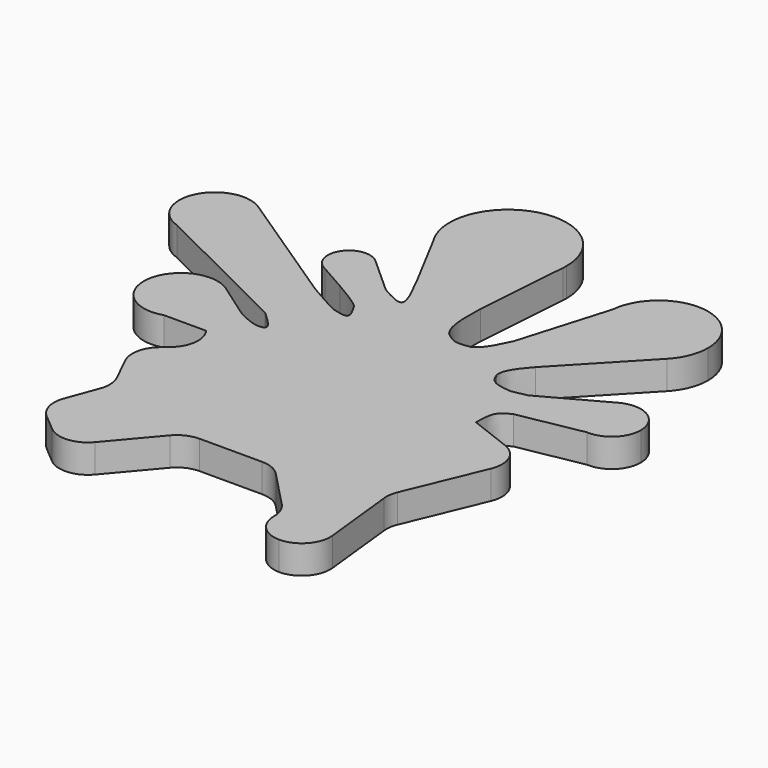
from build123d import *

# Parameters (mm, degrees)
F1_DEPTH     = 5.08
F2_T1_DEPTH  = 30.48
F2_T3_DEPTH  = 33.4016018607
F2_T5_DEPTH  = 31.1738532926
F2_T7_DEPTH  = 22.9008851429
F2_T9_DEPTH  = 24.6924150926
F2_T11_DEPTH = 5.08
F3_T1_DEPTH  = 38.5956513


# Not quite as in the source:
# - a fillet or chamfer that OpenCascade refuses, or shapes differently, is made with other operations: its cross-section is extruded or revolved along the edge and cut away or added


with BuildPart() as f1:
    # F0 (on Top) → F1 (new body)
    with BuildSketch(Plane.XY):
        with BuildLine():
            ThreePointArc((-21.5558748819, 0), (0, -21.5558748819), (21.5558748819, 0))
            ThreePointArc((21.5558748819, 0), (21.4234709168, 2.3855053553), (21.0278855675, 4.7417054405))
            ThreePointArc((21.0278855675, 4.7417054405), (20.3885232844, 6.9974181101), (19.5079583491, 9.1703491196))
            ThreePointArc((19.5079583491, 9.1703491196), (18.4039292813, 11.2227950589), (17.0847745632, 13.1440564533))
            ThreePointArc((17.0847745632, 13.1440564533), (16.1728801059, 14.2510943792), (15.1893864462, 15.2950410693))
            ThreePointArc((15.1893864462, 15.2950410693), (13.7642148433, 16.5892173315), (12.2292624666, 17.7510811346))
            ThreePointArc((12.2292624666, 17.7510811346), (10.0743632522, 19.0568346529), (7.7818181976, 20.102214989))
            ThreePointArc((7.7818181976, 20.102214989), (5.7045723263, 20.7873422182), (3.5685890575, 21.2584315993))
            ThreePointArc((3.5685890575, 21.2584315993), (1.5124623044, 21.5027486546), (-0.5576198391, 21.5486612586))
            ThreePointArc((-0.5576198391, 21.5486612586), (-3.1118074322, 21.3300819602), (-5.6219845653, 20.8098301644))
            Line((-5.6219845653, 20.8098301644), (-9.4810400544, 19.3588641561))
            ThreePointArc((-9.4810400544, 19.3588641561), (-10.7139746116, 18.7047183872), (-11.9019916348, 17.972154491))
            ThreePointArc((-11.9019916348, 17.972154491), (-12.7090282155, 17.4108111167), (-13.489631919, 16.81325586))
            Line((-13.489631919, 16.81325586), (-18.8732484452, 10.4142323313))
            ThreePointArc((-18.8732484452, 10.4142323313), (-19.2769960016, 9.6464069518), (-19.6495220596, 8.8629580138))
            add(Edge.make_bspline(
                [(-19.689484951, 8.773820393), (-19.671758168, 8.8014219328), (-19.6583090598, 8.8311154874), (-19.6495220596, 8.8629580138)],
                knots=[0.5880065236, 0.5880065236, 0.5880065236, 0.5880065236, 0.6086967417, 0.6086967417, 0.6086967417, 0.6086967417], degree=3))
            ThreePointArc((-19.689484951, 8.773820393), (-20.0824369178, 7.8327178788), (-20.4304363673, 6.8740826127))
            ThreePointArc((-20.4304363673, 6.8740826127), (-20.9968993757, 4.8770850443), (-21.3686524004, 2.834860934))
            ThreePointArc((-21.3686524004, 2.834860934), (-21.5090183349, 1.4205182833), (-21.5558748819, 0))
        make_face()
        with BuildLine():
            ThreePointArc((21.0278855675, 4.7417054405), (21.4234709168, 2.3855053553), (21.5558748819, 0))
            ThreePointArc((21.5558748819, 0), (0, -21.5558748819), (-21.5558748819, 0))
            Line((-21.5558748819, 0), (-30.4278861731, -7.6231318526))
            Line((-30.4278861731, -7.6231318526), (-25.4074353725, -17.9089326411))
            Line((-25.4074353725, -17.9089326411), (-29.4482856989, -28.8069844246))
            Line((-29.4482856989, -28.8069844246), (-19.897185266, -36.8886850774))
            Line((-19.897185266, -36.8886850774), (-8.2437438999, -23.1164366785))
            Line((-8.2437438999, -23.1164366785), (7.4091665447, -23.1164366785))
            Line((7.4091665447, -23.1164366785), (17.6949668676, -33.8274315))
            Line((17.6949668676, -33.8274315), (15.0010669604, -39.9499349296))
            Line((15.0010669604, -39.9499349296), (27.3685175925, -39.9499349296))
            Line((27.3685175925, -39.9499349296), (25.1644179225, -19.7456832975))
            Line((25.1644179225, -19.7456832975), (33.3685651422, 0))
            Line((33.3685651422, 0), (21.0278855675, 4.7417054405))
        make_face()
        with BuildLine():
            ThreePointArc((19.5079583491, 9.1703491196), (20.3885232844, 6.9974181101), (21.0278855675, 4.7417054405))
            add(Edge.make_bspline(
                [(23.5232420106, 9.9174740822), (22.7559455678, 9.5391724766), (21.0414634986, 8.6938781634), (21.0327174333, 6.1481323969), (21.0278855675, 4.7417054405)],
                knots=[0, 0, 0, 0, 0.4475383305, 1, 1, 1, 1], degree=3))
            Line((23.5232420106, 9.9174740822), (19.5079583491, 9.1703491196))
        make_face()
        with BuildLine():
            add(Edge.make_bspline(
                [(-25.5037302423, 2.834860934), (-24.5160973645, 2.5129693408), (-22.6879107249, 1.9171225202), (-21.9124239812, 0.6038221422), (-21.5558748819, 0)],
                knots=[0, 0, 0, 0, 0.5402254105, 1, 1, 1, 1], degree=3))
            ThreePointArc((-21.5558748819, 0), (-21.5090183349, 1.4205182833), (-21.3686524004, 2.834860934))
            Line((-21.3686524004, 2.834860934), (-25.5037302423, 2.834860934))
        make_face()
        with BuildLine():
            ThreePointArc((17.0847745632, 13.1440564533), (18.4039292813, 11.2227950589), (19.5079583491, 9.1703491196))
            Line((19.5079583491, 9.1703491196), (23.5232420106, 9.9174740822))
            Line((23.5232420106, 9.9174740822), (34.937579099, 12.0413430014))
            ThreePointArc((34.937579099, 12.0413430014), (30.2244051694, 16.0664474688), (32.7872119933, 21.7098060121))
            Line((32.7872119933, 21.7098060121), (21.5822452322, 15.5974467356))
            Line((21.5822452322, 15.5974467356), (21.0278855675, 15.2950410693))
            Line((21.0278855675, 15.2950410693), (17.0847745632, 13.1440564533))
        make_face()
        with BuildLine():
            Line((-25.5037302423, 2.834860934), (-21.3686524004, 2.834860934))
            ThreePointArc((-21.3686524004, 2.834860934), (-20.9968993757, 4.8770850443), (-20.4304363673, 6.8740826127))
            Line((-20.4304363673, 6.8740826127), (-24.9308068167, 10.0250903474))
            Line((-24.9308068167, 10.0250903474), (-30.9927849426, 14.269483154))
            ThreePointArc((-30.9927849426, 14.269483154), (-29.1301786272, 11.9719193672), (-28.4643126696, 9.0901275345))
            ThreePointArc((-28.4643126696, 9.0901275345), (-29.7263545066, 5.2187104583), (-33.0275484153, 2.834860934))
            Line((-33.0275484153, 2.834860934), (-25.5037302423, 2.834860934))
        make_face()
        with BuildLine():
            ThreePointArc((15.1893864462, 15.2950410693), (16.1728801059, 14.2510943792), (17.0847745632, 13.1440564533))
            Line((17.0847745632, 13.1440564533), (21.0278855675, 15.2950410693))
            Line((21.0278855675, 15.2950410693), (21.5822452322, 15.5974467356))
            add(Edge.make_bspline(
                [(21.5822452322, 15.5974467356), (20.6461265257, 15.3814646696), (19.7100078192, 15.1654826036), (18.8297399827, 15.0541492613)],
                knots=[0, 0, 0, 0, 0.3951796339, 0.3951796339, 0.3951796339, 0.3951796339], degree=3))
            add(Edge.make_bspline(
                [(18.8297399827, 15.0541492613), (18.5066864561, 15.0132905279), (17.1908116294, 14.9016748686), (16.0537750645, 15.1251514978), (15.1893864462, 15.2950410693)],
                knots=[0.3951796339, 0.3951796339, 0.3951796339, 0.3951796339, 0.5402084184, 1, 1, 1, 1], degree=3))
        make_face()
        with BuildLine():
            ThreePointArc((32.7872119933, 21.7098060121), (30.2244051694, 16.0664474688), (34.937579099, 12.0413430014))
            ThreePointArc((34.937579099, 12.0413430014), (38.7854990971, 13.4304076429), (40.4091437753, 17.1853732684))
            ThreePointArc((40.4091437753, 17.1853732684), (37.8860736917, 21.6171995213), (32.7872119933, 21.7098060121))
        make_face()
        with BuildLine():
            Line((-24.9308068167, 10.0250903474), (-20.4304363673, 6.8740826127))
            ThreePointArc((-20.4304363673, 6.8740826127), (-20.0824369178, 7.8327178788), (-19.689484951, 8.773820393))
            add(Edge.make_bspline(
                [(-24.9308068167, 10.0250903474), (-23.6422724453, 9.3599481679), (-21.6239700291, 8.3165515966), (-19.8715548677, 8.4903278918), (-19.689484951, 8.773820393)],
                knots=[0, 0, 0, 0, 0.3754994773, 0.5880065236, 0.5880065236, 0.5880065236, 0.5880065236], degree=3))
        make_face()
        with BuildLine():
            ThreePointArc((-31.5485147848, 14.6585864624), (-41.5514457727, 9.9054871575), (-33.0275484153, 2.834860934))
            ThreePointArc((-33.0275484153, 2.834860934), (-29.7263545066, 5.2187104583), (-28.4643126696, 9.0901275345))
            ThreePointArc((-28.4643126696, 9.0901275345), (-29.1301786272, 11.9719193672), (-30.9927849426, 14.269483154))
            Line((-30.9927849426, 14.269483154), (-31.5485147848, 14.6585864624))
        make_face()
        with BuildLine():
            add(Edge.make_bspline(
                [(14.372244753, 17.5998769298), (14.4881018562, 16.8222590075), (14.8387441512, 16.0586500384), (15.1893864462, 15.2950410693)],
                knots=[0.6845639483, 0.6845639483, 0.6845639483, 0.6845639483, 1, 1, 1, 1], degree=3))
            add(Edge.make_bspline(
                [(18.8297399827, 15.0541492613), (18.5066864561, 15.0132905279), (17.1908116294, 14.9016748686), (16.0537750645, 15.1251514978), (15.1893864462, 15.2950410693)],
                knots=[0.3951796339, 0.3951796339, 0.3951796339, 0.3951796339, 0.5402084184, 1, 1, 1, 1], degree=3))
            add(Edge.make_bspline(
                [(14.372244753, 17.5998769298), (14.6351603968, 16.9655355449), (15.2435298304, 15.5008816531), (17.5314333381, 15.2122461299), (18.8297399827, 15.0541492613)],
                knots=[0, 0, 0, 0, 0.4324268759, 1, 1, 1, 1], degree=3))
        make_face()
        with BuildLine():
            ThreePointArc((12.2292624666, 17.7510811346), (13.7642148433, 16.5892173315), (15.1893864462, 15.2950410693))
            add(Edge.make_bspline(
                [(14.372244753, 17.5998769298), (14.4881018562, 16.8222590075), (14.8387441512, 16.0586500384), (15.1893864462, 15.2950410693)],
                knots=[0.6845639483, 0.6845639483, 0.6845639483, 0.6845639483, 1, 1, 1, 1], degree=3))
            add(Edge.make_bspline(
                [(17.0847745632, 22.8695263715), (15.8418994446, 21.4312290193), (14.2906498457, 19.6360702318), (14.3222617771, 17.9353562123), (14.372244753, 17.5998769298)],
                knots=[0, 0, 0, 0, 0.548478787, 0.6845639483, 0.6845639483, 0.6845639483, 0.6845639483], degree=3))
            Line((17.0847745632, 22.8695263715), (12.2292624666, 17.7510811346))
        make_face()
        with BuildLine():
            ThreePointArc((-19.6495220596, 8.8629580138), (-19.6695539991, 8.8184118412), (-19.689484951, 8.773820393))
            add(Edge.make_bspline(
                [(-19.689484951, 8.773820393), (-19.671758168, 8.8014219328), (-19.6583090598, 8.8311154874), (-19.6495220596, 8.8629580138)],
                knots=[0.5880065236, 0.5880065236, 0.5880065236, 0.5880065236, 0.6086967417, 0.6086967417, 0.6086967417, 0.6086967417], degree=3))
        make_face()
        with BuildLine():
            ThreePointArc((-30.9927849426, 14.269483154), (-31.2656234469, 14.4712136982), (-31.5485147848, 14.6585864624))
            Line((-31.5485147848, 14.6585864624), (-30.9927849426, 14.269483154))
        make_face()
        with BuildLine():
            ThreePointArc((7.7818181976, 20.102214989), (10.0743632522, 19.0568346529), (12.2292624666, 17.7510811346))
            Line((12.2292624666, 17.7510811346), (17.0847745632, 22.8695263715))
            Line((17.0847745632, 22.8695263715), (29.8265086684, 36.3012441684))
            ThreePointArc((29.8265086684, 36.3012441684), (19.7700953097, 34.3405012918), (14.6350970936, 43.2066027795))
            Line((14.6350970936, 43.2066027795), (9.8595311749, 27.1067871176))
            Line((9.8595311749, 27.1067871176), (7.7818181976, 20.102214989))
        make_face()
        with BuildLine():
            add(Edge.make_bspline(
                [(-19.6495220596, 8.8629580138), (-19.4833381268, 9.4651790358), (-20.9847051533, 10.8360480358), (-22.495258138, 12.2115954812)],
                knots=[0.6086967417, 0.6086967417, 0.6086967417, 0.6086967417, 1, 1, 1, 1], degree=3))
            ThreePointArc((-19.6495220596, 8.8629580138), (-19.2769960016, 9.6464069518), (-18.8732484452, 10.4142323313))
            Line((-18.8732484452, 10.4142323313), (-22.495258138, 12.2115954812))
        make_face()
        with BuildLine():
            ThreePointArc((3.5685890575, 21.2584315993), (5.7045723263, 20.7873422182), (7.7818181976, 20.102214989))
            Line((7.7818181976, 20.102214989), (9.8595311749, 27.1067871176))
            add(Edge.make_bspline(
                [(9.8595311749, 27.1067871176), (9.0003739191, 25.2647119406), (7.9917320333, 23.0991990151), (6.5049700197, 22.1455177099), (6.2757189942, 22.0247046239)],
                knots=[0, 0, 0, 0, 0.553515968, 0.6501455724, 0.6501455724, 0.6501455724, 0.6501455724], degree=3))
            add(Edge.make_bspline(
                [(6.2757189942, 22.0247046239), (5.4456991801, 21.5872921634), (4.5071787847, 21.424245643), (3.5685890575, 21.2584315993)],
                knots=[0.6501455724, 0.6501455724, 0.6501455724, 0.6501455724, 1, 1, 1, 1], degree=3))
        make_face()
        with BuildLine():
            Line((-22.495258138, 12.2115954812), (-18.8732484452, 10.4142323313))
            ThreePointArc((-18.8732484452, 10.4142323313), (-16.49472285, 13.8773145827), (-13.489631919, 16.81325586))
            Line((-13.489631919, 16.81325586), (-21.4981341047, 22.1309257933))
            Line((-21.4981341047, 22.1309257933), (-43.1270560205, 36.4925960649))
            ThreePointArc((-43.1270560205, 36.4925960649), (-41.0437760026, 34.2040473217), (-40.2896412796, 31.2025823789))
            ThreePointArc((-40.2896412796, 31.2025823789), (-42.8993068164, 26.0710720648), (-48.5833099737, 25.1573650952))
            Line((-48.5833099737, 25.1573650952), (-22.495258138, 12.2115954812))
        make_face()
        with BuildLine():
            add(Edge.make_bspline(
                [(1.4428020951, 23.2494519066), (2.0356785994, 22.4625958954), (2.8021338285, 21.8605137474), (3.5685890575, 21.2584315993)],
                knots=[0.6978886874, 0.6978886874, 0.6978886874, 0.6978886874, 1, 1, 1, 1], degree=3))
            add(Edge.make_bspline(
                [(6.2757189942, 22.0247046239), (5.4456991801, 21.5872921634), (4.5071787847, 21.424245643), (3.5685890575, 21.2584315993)],
                knots=[0.6501455724, 0.6501455724, 0.6501455724, 0.6501455724, 1, 1, 1, 1], degree=3))
            add(Edge.make_bspline(
                [(1.4428020951, 23.2494519066), (2.1136741264, 22.6899001143), (3.4684392223, 21.5687785752), (5.3321614448, 21.8612087878), (6.2757189942, 22.0247046239)],
                knots=[0, 0, 0, 0, 0.4858514557, 0.9775111942, 0.9775111942, 0.9775111942, 0.9775111942], degree=3))
        make_face()
        with BuildLine():
            ThreePointArc((-0.5576198391, 21.5486612586), (1.5124623044, 21.5027486546), (3.5685890575, 21.2584315993))
            add(Edge.make_bspline(
                [(1.4428020951, 23.2494519066), (2.0356785994, 22.4625958954), (2.8021338285, 21.8605137474), (3.5685890575, 21.2584315993)],
                knots=[0.6978886874, 0.6978886874, 0.6978886874, 0.6978886874, 1, 1, 1, 1], degree=3))
            add(Edge.make_bspline(
                [(0.1873508122, 31.7397286266), (0.1000880741, 28.9584711756), (-0.0062348151, 25.5697243407), (1.1972842983, 23.5752991157), (1.4428020951, 23.2494519066)],
                knots=[0, 0, 0, 0, 0.5727805016, 0.6978886874, 0.6978886874, 0.6978886874, 0.6978886874], degree=3))
            Line((0.1873508122, 31.7397286266), (-0.5576198391, 21.5486612586))
        make_face()
        with BuildLine():
            ThreePointArc((14.6350970936, 43.2066027795), (19.7700953097, 34.3405012918), (29.8265086684, 36.3012441684))
            ThreePointArc((29.8265086684, 36.3012441684), (31.6214054529, 39.1059647688), (32.2495003028, 42.3760731726))
            ThreePointArc((32.2495003028, 42.3760731726), (23.8384448664, 51.1930593335), (14.6350970936, 43.2066027795))
        make_face()
        with BuildLine():
            Line((-21.4981341047, 22.1309257933), (-13.489631919, 16.81325586))
            ThreePointArc((-13.489631919, 16.81325586), (-12.7090282155, 17.4108111167), (-11.9019916348, 17.972154491))
            add(Edge.make_bspline(
                [(-15.6037653952, 18.9190625193), (-15.1517196516, 18.7132722351), (-13.629732374, 18.0898022553), (-12.6272962109, 18.0215429553), (-11.9019916348, 17.972154491)],
                knots=[0.5064082285, 0.5064082285, 0.5064082285, 0.5064082285, 0.6428656669, 1, 1, 1, 1], degree=3))
            add(Edge.make_bspline(
                [(-21.4981341047, 22.1309257933), (-19.3897449339, 20.9068490942), (-17.2813557631, 19.682772395), (-15.6037653952, 18.9190625193)],
                knots=[0, 0, 0, 0, 0.5064082285, 0.5064082285, 0.5064082285, 0.5064082285], degree=3))
        make_face()
        with BuildLine():
            ThreePointArc((-43.1270560205, 36.4925960649), (-52.3612879028, 33.9567174372), (-48.5833099737, 25.1573650952))
            ThreePointArc((-48.5833099737, 25.1573650952), (-42.8993068164, 26.0710720648), (-40.2896412796, 31.2025823789))
            ThreePointArc((-40.2896412796, 31.2025823789), (-41.0437760026, 34.2040473217), (-43.1270560205, 36.4925960649))
        make_face()
        with BuildLine():
            ThreePointArc((-5.6219845653, 20.8098301644), (-3.1118074322, 21.3300819602), (-0.5576198391, 21.5486612586))
            Line((-0.5576198391, 21.5486612586), (0.1873508122, 31.7397286266))
            Line((0.1873508122, 31.7397286266), (1.4229034066, 48.6418706156))
            ThreePointArc((1.4229034066, 48.6418706156), (-6.4142835546, 39.2859820381), (-17.7701736912, 43.7578842893))
            Line((-17.7701736912, 43.7578842893), (-12.108076115, 33.0621237696))
            Line((-12.108076115, 33.0621237696), (-5.6219845653, 20.8098301644))
        make_face()
        with BuildLine():
            add(Edge.make_bspline(
                [(-14.1186807086, 21.5523049049), (-13.7674127143, 21.2535588061), (-12.528919888, 20.0549599754), (-12.1730615765, 18.869117359), (-11.9019916348, 17.972154491)],
                knots=[0.4851885937, 0.4851885937, 0.4851885937, 0.4851885937, 0.6132384939, 1, 1, 1, 1], degree=3))
            ThreePointArc((-11.9019916348, 17.972154491), (-10.7139746116, 18.7047183872), (-9.4810400544, 19.3588641561))
            Line((-9.4810400544, 19.3588641561), (-19.3532919722, 24.9653740527))
            add(Edge.make_bspline(
                [(-19.3532919722, 24.9653740527), (-17.4010758423, 23.8250906074), (-15.4496557731, 22.6842714218), (-14.1186807086, 21.5523049049)],
                knots=[0, 0, 0, 0, 0.4851885937, 0.4851885937, 0.4851885937, 0.4851885937], degree=3))
        make_face()
        with BuildLine():
            add(Edge.make_bspline(
                [(-15.6037653952, 18.9190625193), (-15.1517196516, 18.7132722351), (-13.629732374, 18.0898022553), (-12.6272962109, 18.0215429553), (-11.9019916348, 17.972154491)],
                knots=[0.5064082285, 0.5064082285, 0.5064082285, 0.5064082285, 0.6428656669, 1, 1, 1, 1], degree=3))
            add(Edge.make_bspline(
                [(-14.1186807086, 21.5523049049), (-13.7674127143, 21.2535588061), (-12.528919888, 20.0549599754), (-12.1730615765, 18.869117359), (-11.9019916348, 17.972154491)],
                knots=[0.4851885937, 0.4851885937, 0.4851885937, 0.4851885937, 0.6132384939, 1, 1, 1, 1], degree=3))
            add(Edge.make_bspline(
                [(-15.6037653952, 18.9190625193), (-14.4283120532, 18.5905868682), (-11.9718187149, 17.9265406092), (-13.3807906918, 20.3143200715), (-14.1186807086, 21.5523049049)],
                knots=[0, 0, 0, 0, 0.4799231847, 1, 1, 1, 1], degree=3))
        make_face()
        with BuildLine():
            ThreePointArc((-9.4810400544, 19.3588641561), (-7.5862812863, 20.1768203186), (-5.6219845653, 20.8098301644))
            Line((-5.6219845653, 20.8098301644), (-13.7229076454, 28.1006093155))
            Line((-13.7229076454, 28.1006093155), (-20.2650786975, 33.9885215741))
            ThreePointArc((-20.2650786975, 33.9885215741), (-19.348532067, 32.7274543218), (-19.0243201626, 31.2025822021))
            ThreePointArc((-19.0243201626, 31.2025822021), (-20.7539962478, 28.0443911329), (-24.3465941192, 27.8010996944))
            Line((-24.3465941192, 27.8010996944), (-19.3532919722, 24.9653740527))
            Line((-19.3532919722, 24.9653740527), (-9.4810400544, 19.3588641561))
        make_face()
        with BuildLine():
            Line((-13.7229076454, 28.1006093155), (-5.6219845653, 20.8098301644))
            Line((-5.6219845653, 20.8098301644), (-12.108076115, 33.0621237696))
            add(Edge.make_bspline(
                [(-12.108076115, 33.0621237696), (-10.5611501023, 30.0773195503), (-7.7878381604, 24.7261953741), (-11.9030987649, 27.065947721), (-13.7229076454, 28.1006093155)],
                knots=[0, 0, 0, 0, 0.5577901243, 1, 1, 1, 1], degree=3))
        make_face()
        with BuildLine():
            ThreePointArc((-17.7701736912, 43.7578842893), (-6.4142835546, 39.2859820381), (1.4229034066, 48.6418706156))
            ThreePointArc((1.4229034066, 48.6418706156), (1.4437368542, 49.022163574), (1.4506844192, 49.4029633877))
            ThreePointArc((1.4506844192, 49.4029633877), (-11.0750760863, 59.6317500163), (-18.5941676648, 45.3144173747))
            Line((-18.5941676648, 45.3144173747), (-17.7701736912, 43.7578842893))
        make_face()
        with BuildLine():
            ThreePointArc((-19.0243201626, 31.2025822021), (-19.348532067, 32.7274543218), (-20.2650786975, 33.9885215741))
            ThreePointArc((-20.2650786975, 33.9885215741), (-25.9011017814, 33.2664173148), (-24.3465941192, 27.8010996944))
            ThreePointArc((-24.3465941192, 27.8010996944), (-20.7539962478, 28.0443911329), (-19.0243201626, 31.2025822021))
        make_face()
        with BuildLine():
            ThreePointArc((-18.5941676648, 45.3144173747), (-18.215053705, 44.5187432893), (-17.7701736912, 43.7578842893))
            Line((-17.7701736912, 43.7578842893), (-18.5941676648, 45.3144173747))
        make_face()
        with BuildLine():
            ThreePointArc((-13.489631919, 16.81325586), (-16.49472285, 13.8773145827), (-18.8732484452, 10.4142323313))
            Line((-18.8732484452, 10.4142323313), (-13.489631919, 16.81325586))
        make_face()
        with BuildLine():
            Line((-9.4810400544, 19.3588641561), (-5.6219845653, 20.8098301644))
            ThreePointArc((-5.6219845653, 20.8098301644), (-7.5862812863, 20.1768203186), (-9.4810400544, 19.3588641561))
        make_face()
    extrude(amount=F1_DEPTH)

    # F2: fillet of radius 5.08 on 11 edges, made by hand

    # F2_s2 → F2_t1 (cut)
    with BuildSketch(Plane.XY.offset(-12.7)):
        with BuildLine():
            ThreePointArc((-23.7751875383, -33.607298423), (-20.0719299347, -34.7917486099), (-16.6157986116, -33.0106828051))
            Line((-16.6157986116, -33.0106828051), (-16.5382385661, -33.0763105382))
            Line((-16.5382385661, -33.0763105382), (-19.8852529537, -37.031872856))
            Line((-19.8852529537, -37.031872856), (-23.8408152714, -33.6848584684))
            Line((-23.8408152714, -33.6848584684), (-23.7751875383, -33.607298423))
        make_face()
    extrude(amount=F2_T1_DEPTH, mode=Mode.SUBTRACT)

    # F2_s4 → F2_t3 (cut)
    with BuildSketch(Plane.XY.offset(-14.1608009303)):
        with BuildLine():
            ThreePointArc((21.7041972204, -39.9499349296), (25.4860644305, -38.2616720075), (26.7542362913, -34.3190217034))
            Line((26.7542362913, -34.3190217034), (26.8552370727, -34.3080034389))
            Line((26.8552370727, -34.3080034389), (27.481804, -40.0515349296))
            Line((27.481804, -40.0515349296), (21.7041972204, -40.0515349296))
            Line((21.7041972204, -40.0515349296), (21.7041972204, -39.9499349296))
        make_face()
    extrude(amount=F2_T3_DEPTH, mode=Mode.SUBTRACT)

    # F2_s6 → F2_t5 (cut)
    with BuildSketch(Plane.XY.offset(-13.0469266463)):
        with BuildLine():
            ThreePointArc((31.3661757916, -4.8193364766), (31.3438624437, -0.8681884219), (28.4970258172, 1.8718097639))
            Line((28.4970258172, 1.8718097639), (28.5334665587, 1.9666497995))
            Line((28.5334665587, 1.9666497995), (33.5024366701, 0.0574038404))
            Line((33.5024366701, 0.0574038404), (31.4599995324, -4.8583193657))
            Line((31.4599995324, -4.8583193657), (31.3661757916, -4.8193364766))
        make_face()
    extrude(amount=F2_T5_DEPTH, mode=Mode.SUBTRACT)

    # F2_s8 → F2_t7 (cut)
    with BuildSketch(Plane.XY.offset(-8.9104425714)):
        with BuildLine():
            ThreePointArc((-28.2091730806, -25.465134965), (-28.3595555101, -28.5211629615), (-26.7274418769, -31.109236971))
            Line((-26.7274418769, -31.109236971), (-26.79306961, -31.1867970164))
            Line((-26.79306961, -31.1867970164), (-29.5683303084, -28.8384994191))
            Line((-29.5683303084, -28.8384994191), (-28.3044354378, -25.4298129704))
            Line((-28.3044354378, -25.4298129704), (-28.2091730806, -25.465134965))
        make_face()
    extrude(amount=F2_T7_DEPTH, mode=Mode.SUBTRACT)

    # F2_s10 → F2_t9 (cut)
    with BuildSketch(Plane.XY.offset(-9.8062075463)):
        with BuildLine():
            ThreePointArc((-27.4527909667, -5.0668295342), (-29.1173620778, -7.8934900279), (-28.7073500706, -11.1481323562))
            Line((-28.7073500706, -11.1481323562), (-28.7986544942, -11.1926976143))
            Line((-28.7986544942, -11.1926976143), (-30.5536013188, -7.5971971006))
            Line((-30.5536013188, -7.5971971006), (-27.5190042082, -4.9897687358))
            Line((-27.5190042082, -4.9897687358), (-27.4527909667, -5.0668295342))
        make_face()
    extrude(amount=F2_T9_DEPTH, mode=Mode.SUBTRACT)

    # F2_s12 → F2_t11 (join)
    with BuildSketch(Plane.XY):
        with BuildLine():
            ThreePointArc((-5.8876452816, -23.1164366785), (-8.0250450799, -23.587974668), (-9.7656475539, -24.915050024))
            Line((-9.7656475539, -24.915050024), (-9.8432075993, -24.8494222909))
            Line((-9.8432075993, -24.8494222909), (-8.2908658722, -23.0148366785))
            Line((-8.2908658722, -23.0148366785), (-5.8876452816, -23.0148366785))
            Line((-5.8876452816, -23.0148366785), (-5.8876452816, -23.1164366785))
        make_face()
        with BuildLine():
            ThreePointArc((8.9085458148, -24.6777973012), (7.2358985953, -23.523049896), (5.2444528939, -23.1164366785))
            Line((5.2444528939, -23.1164366785), (5.2444528939, -23.0148366785))
            Line((5.2444528939, -23.0148366785), (7.4524608177, -23.0148366785))
            Line((7.4524608177, -23.0148366785), (8.9818276732, -24.6074245137))
            Line((8.9818276732, -24.6074245137), (8.9085458148, -24.6777973012))
        make_face()
        with BuildLine():
            ThreePointArc((25.6646602449, -18.5417036265), (25.3273839394, -19.7690750319), (25.3058082185, -21.0417613096))
            Line((25.3058082185, -21.0417613096), (25.2048074371, -21.0527795742))
            Line((25.2048074371, -21.0527795742), (25.0605893352, -19.7307800018))
            Line((25.0605893352, -19.7307800018), (25.570836504, -18.5027207374))
            Line((25.570836504, -18.5027207374), (25.6646602449, -18.5417036265))
        make_face()
        with BuildLine():
            ThreePointArc((-26.1636731936, -19.9484832976), (-25.8530143, -17.9310084007), (-26.3615698708, -15.9541206601))
            Line((-26.3615698708, -15.9541206601), (-26.2702654472, -15.909555402))
            Line((-26.2702654472, -15.909555402), (-25.2970482589, -17.9034636227))
            Line((-25.2970482589, -17.9034636227), (-26.0684108365, -19.9838052922))
            Line((-26.0684108365, -19.9838052922), (-26.1636731936, -19.9484832976))
        make_face()
        with BuildLine():
            ThreePointArc((-26.2692397475, -4.049882339), (-24.531015773, -0.7582243213), (-25.5037302423, 2.834860934))
            Line((-25.5037302423, 2.834860934), (-25.4222068107, 2.8954950011))
            ThreePointArc((-25.4222068107, 2.8954950011), (-23.1778893513, 2.0067211174), (-21.468388576, 0.0516595226))
            Line((-21.468388576, 0.0516595226), (-21.4896616404, -0.0770607984))
            Line((-21.4896616404, -0.0770607984), (-26.2030265059, -4.1269431374))
            Line((-26.2030265059, -4.1269431374), (-26.2692397475, -4.049882339))
        make_face()
        with BuildLine():
            ThreePointArc((16.3256234208, -36.9395775477), (16.6779484431, -34.0075867675), (15.3399155285, -31.3750270292))
            Line((15.3399155285, -31.3750270292), (15.4131973869, -31.3046542417))
            Line((15.4131973869, -31.3046542417), (17.8153497528, -33.8061068018))
            Line((17.8153497528, -33.8061068018), (16.4186194371, -36.9804957705))
            Line((16.4186194371, -36.9804957705), (16.3256234208, -36.9395775477))
        make_face()
    extrude(amount=F2_T11_DEPTH)

    # F3: fillet of radius 5.08 on 1 edges, made by hand

    # F3_s2 → F3_t1 (cut)
    with BuildSketch(Plane.XY.offset(-16.75782565)):
        with BuildLine():
            ThreePointArc((21.7041972204, -39.9499349296), (18.2013107758, -38.4208506374), (16.7558106694, -34.882653122))
            Line((16.7558106694, -34.882653122), (16.2478118633, -34.8837544504))
            ThreePointArc((16.2478118633, -34.8837544504), (15.8606433395, -36.7349864336), (14.5360868791, -39.7453438155))
            Line((14.5360868791, -39.7453438155), (15.0010669604, -40.4579349296))
            ThreePointArc((15.0010669604, -40.4579349296), (18.3526320904, -40.4579349296), (21.6910370693, -40.4577644388))
            Line((21.6910370693, -40.4577644388), (21.7041972204, -39.9499349296))
        make_face()
    extrude(amount=F3_T1_DEPTH, mode=Mode.SUBTRACT)


solid = f1.part
